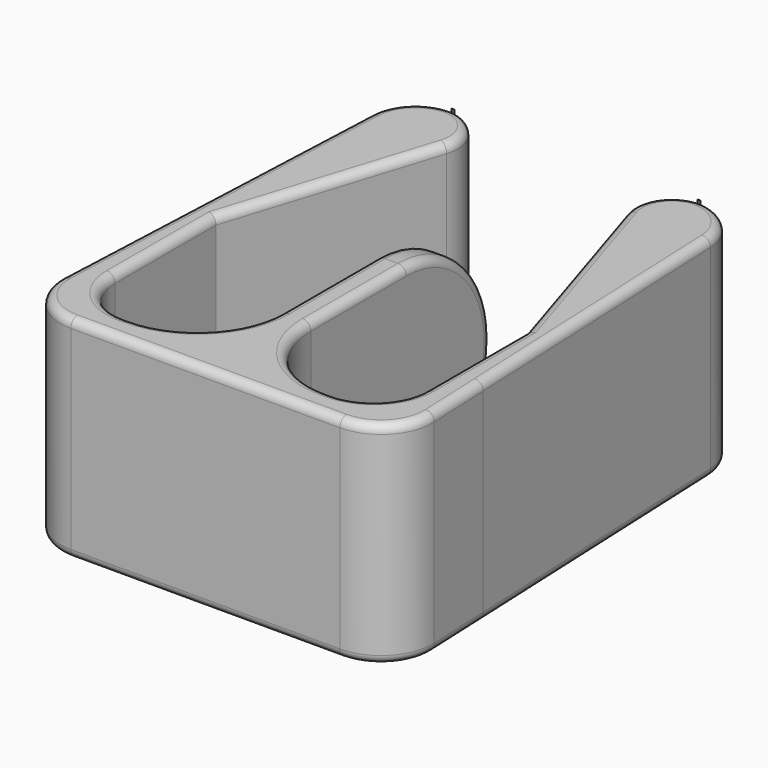
from build123d import *

# Parameters (mm, degrees)
F1_DEPTH = 6.35
F2_R     = 3.17499
F3_R     = 2.5146
F4_R     = 0.254


# Not quite as in the source:
# - a fillet or chamfer is up to 0.001 mm smaller than in the source, because OpenCascade refuses the exact size


with BuildPart() as f1:
    # F0 (on Top) → F1 (new body)
    with BuildSketch(Plane.XY):
        with BuildLine():
            ThreePointArc((-3.693303641, 4.1775837632), (-4.6679721343, 3.794454123), (-5.1024929117, 2.8415854608))
            Line((-5.1024929117, 2.8415854608), (-5.4963516714, -6.179263229))
            Line((-5.4963516714, -6.179263229), (-4.6539532316, -3.5099362281))
            Line((-4.6539532316, -3.5099362281), (-2.6959738617, 2.6943573136))
            ThreePointArc((-2.6959738617, 2.6943573136), (-2.8374693082, 3.6761332742), (-3.693303641, 4.1775837632))
        make_face()
        with BuildLine():
            Line((-4.6539532316, -3.5099362281), (-5.4963516714, -6.179263229))
            Line((-5.4963516714, -6.179263229), (-5.5811456925, -8.1213656104))
            ThreePointArc((-5.5811456925, -8.1213656104), (-5.1539371815, -9.2564313962), (-4.0385863003, -9.7327441736))
            Line((-4.0385863003, -9.7327441736), (0, -9.7327441736))
            Line((0, -9.7327441736), (0, 0.4272558264))
            Line((0, 0.4272558264), (-0.4445, 0.4272558264))
            Line((-0.4445, 0.4272558264), (-0.4445, -8.8437441736))
            Line((-0.4445, -8.8437441736), (-3.1099126316, -8.8437441736))
            ThreePointArc((-3.1099126316, -8.8437441736), (-4.2017142103, -8.3915051523), (-4.6539532316, -7.2997035736))
            Line((-4.6539532316, -7.2997035736), (-4.6539532316, -3.5099362281))
        make_face()
        with BuildLine():
            Line((0, 0.4272558264), (0, -9.7327441736))
            Line((0, -9.7327441736), (4.0385863003, -9.7327441736))
            ThreePointArc((4.0385863003, -9.7327441736), (5.1539371815, -9.2564313962), (5.5811456925, -8.1213656104))
            Line((5.5811456925, -8.1213656104), (5.4963516714, -6.179263229))
            Line((5.4963516714, -6.179263229), (4.6539532316, -3.5099362281))
            Line((4.6539532316, -3.5099362281), (4.6539532316, -7.2997035736))
            ThreePointArc((4.6539532316, -7.2997035736), (4.2017142103, -8.3915051523), (3.1099126316, -8.8437441736))
            Line((3.1099126316, -8.8437441736), (0.4445, -8.8437441736))
            Line((0.4445, -8.8437441736), (0.4445, 0.4272558264))
            Line((0.4445, 0.4272558264), (0, 0.4272558264))
        make_face()
        with BuildLine():
            Line((4.6539532316, -3.5099362281), (5.4963516714, -6.179263229))
            Line((5.4963516714, -6.179263229), (5.1024929117, 2.8415854608))
            ThreePointArc((5.1024929117, 2.8415854608), (4.6679721343, 3.794454123), (3.693303641, 4.1775837632))
            ThreePointArc((3.693303641, 4.1775837632), (2.8374693082, 3.6761332742), (2.6959738617, 2.6943573136))
            Line((2.6959738617, 2.6943573136), (4.6539532316, -3.5099362281))
        make_face()
    extrude(amount=F1_DEPTH)

    # F2 (radius 3.175 in the source; OpenCascade refuses exactly that, so slightly less here)
    f2_edges = [f1.edges().sort_by_distance(p)[0] for p in [
        (0, 0.427256, 6.35),
        (0, 0.427256, 0),
    ]]
    fillet(f2_edges, radius=F2_R)

    # F3
    f3_edges = [f1.edges().sort_by_distance(p)[0] for p in [
        (-0.4445, -8.843744, 3.175),
        (0.4445, -8.843744, 3.175),
    ]]
    fillet(f3_edges, radius=F3_R)

    # F4
    f4_edges = [f1.edges().sort_by_distance(p)[0] for p in [
        (3.674964, -0.407789, 0),
        (5.341819, -2.63989, 0),
        (4.667972, 3.794454, 0),
        (2.837469, 3.676133, 0),
        (4.653953, -5.40482, 0),
        (4.201714, -8.391505, 0),
        (0.4445, -4.538439, 0),
        (1.181009, -8.107235, 0),
        (0, -2.747734, 0),
        (3.034506, -8.843744, 0),
        (-0.4445, -4.538439, 0),
        (-1.181009, -8.107235, 0),
        (-3.034506, -8.843744, 0),
        (-4.201714, -8.391505, 0),
        (-4.653953, -5.40482, 0),
        (-3.674964, -0.407789, 0),
        (-2.837469, 3.676133, 0),
        (5.153937, -9.256431, 0),
        (-4.667972, 3.794454, 0),
        (0, -9.732744, 0),
        (-5.341819, -2.63989, 0),
        (-5.153937, -9.256431, 0),
        (0.4445, -4.538439, 6.35),
        (1.181009, -8.107235, 6.35),
        (0, -2.747734, 6.35),
        (3.034506, -8.843744, 6.35),
        (-0.4445, -4.538439, 6.35),
        (4.201714, -8.391505, 6.35),
        (-1.181009, -8.107235, 6.35),
        (4.653953, -5.40482, 6.35),
        (-3.034506, -8.843744, 6.35),
        (3.674964, -0.407789, 6.35),
        (-4.201714, -8.391505, 6.35),
        (2.837469, 3.676133, 6.35),
        (-4.653953, -5.40482, 6.35),
        (4.667972, 3.794454, 6.35),
        (-3.674964, -0.407789, 6.35),
        (5.341819, -2.63989, 6.35),
        (-2.837469, 3.676133, 6.35),
        (5.153937, -9.256431, 6.35),
        (-4.667972, 3.794454, 6.35),
        (0, -9.732744, 6.35),
        (-5.341819, -2.63989, 6.35),
        (-5.153937, -9.256431, 6.35),
        (0.4445, -0.502677, 0.929933),
        (0.4445, 0.427256, 3.175),
        (0.4445, -0.502677, 5.420067),
        (-0.4445, -0.502677, 0.929933),
        (-0.4445, 0.427256, 3.175),
        (-0.4445, -0.502677, 5.420067),
    ]]
    fillet(f4_edges, radius=F4_R)


with BuildPart() as f1b:
    # F0 (on Top) → F1, piece 2 (new body)
    with BuildSketch(Plane.XY):
        with BuildLine():
            ThreePointArc((-3.7361260011, 4.1802594943), (-3.7147022648, 4.1791225794), (-3.693303641, 4.1775837632))
            ThreePointArc((-3.693303641, 4.1775837632), (-3.6695895854, 4.1771529205), (-3.645886262, 4.1763195422))
            Line((-3.645886262, 4.1763195422), (-3.7361260011, 4.1802594943))
        make_face()
    extrude(amount=F1_DEPTH)


with BuildPart() as f1c:
    # F0 (on Top) → F1, piece 3 (new body)
    with BuildSketch(Plane.XY):
        with BuildLine():
            ThreePointArc((3.645886262, 4.1763195422), (3.6695895854, 4.1771529205), (3.693303641, 4.1775837632))
            ThreePointArc((3.693303641, 4.1775837632), (3.7147022648, 4.1791225794), (3.7361260011, 4.1802594943))
            Line((3.7361260011, 4.1802594943), (3.645886262, 4.1763195422))
        make_face()
    extrude(amount=F1_DEPTH)


solid = Compound([f1.part, f1b.part, f1c.part])
